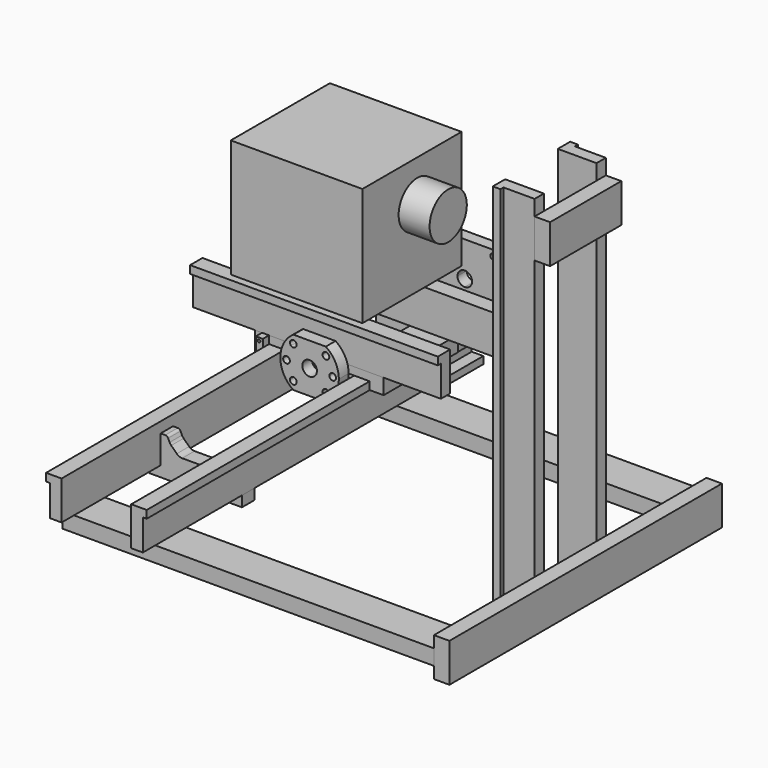
from build123d import *

# Parameters (mm, degrees)
F1_DEPTH       = 304.8
F3_DEPTH       = 76.2
F4_W           = 14.605
F4_H           = 6.35
F5_DEPTH       = 76.2
F7_DEPTH       = 25.4
F7_DEPTH_BACK  = 25.4
F9_DEPTH       = 3.175
F10_DEPTH      = 3.175
F12_DEPTH      = 6.35
F13_DEPTH      = 6.35
F15_DEPTH      = 6.35
F16_R          = 1.190625
F17_DEPTH      = 25.4
F18_DEPTH      = 25.4
F20_DEPTH      = 25.4
F23_DEPTH      = 10
F25_DEPTH      = 32
F27_DEPTH      = 25.4
F29_START      = 63.5
F28_R          = 6
F29_DEPTH      = 25
F30_DEPTH      = 50.8
F31_W          = 32.232244499
F31_H          = 34.175409925
F32_DEPTH      = 101.6
F34_DEPTH      = 50.8
F34_DEPTH_BACK = 152.4
F36_START      = -101.6
F36_DEPTH      = 12.7
F37_W          = 9.525
F37_H          = 5.95
F38_DEPTH      = 38.1
F39_W          = 31.75
F39_H          = 12.7
F40_DEPTH      = 304.8
F42_DEPTH      = 279.4
F44_DEPTH      = 304.8
F46_START      = 28.575
F46_DEPTH      = 9.525
F47_R          = 5.715
F48_DEPTH      = 3.175
F49_W          = 12.7
F49_H          = 31.75
F50_DEPTH      = 73.025
F51_W          = 107.9776808619
F51_H          = 96.8943238258
F52_DEPTH      = 101.6
F53_R          = 19.0804487929
F54_DEPTH      = 25.4


with BuildPart() as f1:
    # F0 (on Front) → F1 (new body)
    with BuildSketch(Plane.XZ):
        Polygon((-38.1, 25.4), (-38.1, 0), (-28.575, 0), (-28.575, 31.75), (-41.275, 31.75), (-41.275, 25.4), align=None)
    extrude(amount=F1_DEPTH)


with BuildPart() as f1b:
    # F0 (on Front) → F1, piece 2 (new body)
    with BuildSketch(Plane.XZ):
        Polygon((28.575, 31.75), (28.575, 0), (38.1, 0), (38.1, 25.4), (41.275, 25.4), (41.275, 31.75), align=None)
    extrude(amount=F1_DEPTH)


with BuildPart() as f3:
    # F2 (on face) → F3 (new body)
    with BuildSketch(Plane(origin=(0, 0, 0), x_dir=(-1, 0, 0), z_dir=(0, 1, 0))):
        Polygon((20.955, 31.75), (28.575, 31.75), (41.275, 31.75), (41.275, 25.4), (52.705, 25.4), (52.705, 38.1), (20.955, 38.1), align=None)
    extrude(amount=-F3_DEPTH)


with BuildPart() as f3b:
    # F2 (on face) → F3, piece 2 (new body)
    with BuildSketch(Plane(origin=(0, 0, 0), x_dir=(-1, 0, 0), z_dir=(0, 1, 0))):
        Polygon((-20.955, 31.75), (-20.955, 38.1), (-52.705, 38.1), (-52.705, 25.4), (-41.275, 25.4), (-41.275, 31.75), (-28.575, 31.75), align=None)
    extrude(amount=-F3_DEPTH)


with BuildPart() as f5:
    # F4 (on face) → F5 (new body)
    with BuildSketch(Plane(origin=(0, 0, 0), x_dir=(-1, 0, 0), z_dir=(0, 1, 0))):
        with Locations((45.4025, 22.225)):
            Rectangle(F4_W, F4_H)
    extrude(amount=-F5_DEPTH)


with BuildPart() as f7_tool:
    # F6 (on face) → F7 (new body, two sides)
    with BuildSketch(Plane(origin=(0, 0, 25.4), x_dir=(1, 0, 0), z_dir=(0, 0, -1))) as f7_sk:
        with BuildLine():
            ThreePointArc((-49.53, 6.35), (-51.1175, 4.7625), (-49.53, 3.175))
            Line((-49.53, 3.175), (-49.53, 6.35))
        make_face()
        with BuildLine():
            ThreePointArc((-49.53, 73.025), (-51.1175, 71.4375), (-49.53, 69.85))
            Line((-49.53, 69.85), (-49.53, 73.025))
        make_face()
        with BuildLine():
            Line((-49.53, 73.025), (-49.53, 69.85))
            ThreePointArc((-49.53, 69.85), (-48.4074679849, 70.3149679849), (-47.9425, 71.4375))
            ThreePointArc((-47.9425, 71.4375), (-48.4074679849, 72.5600320151), (-49.53, 73.025))
        make_face()
        with BuildLine():
            Line((-49.53, 6.35), (-49.53, 3.175))
            ThreePointArc((-49.53, 3.175), (-48.4074679849, 3.6399679849), (-47.9425, 4.7625))
            ThreePointArc((-47.9425, 4.7625), (-48.4074679849, 5.8850320151), (-49.53, 6.35))
        make_face()
    extrude(amount=-F7_DEPTH)
    extrude(f7_sk.sketch, amount=F7_DEPTH_BACK)


with BuildPart() as f3_1:
    add(f3.part)

    # F7: cut by f7_tool
    add(f7_tool.part, mode=Mode.SUBTRACT)

    # F11 (on face) → F12 (cut)
    with BuildSketch(Plane(origin=(0, 0, 25.4), x_dir=(1, 0, 0), z_dir=(0, 0, -1))):
        Polygon((-41.275, 0), (-41.275, 76.2), (-45.2059626353, 76.2), (-42.545, 0), align=None)
    extrude(amount=-F12_DEPTH, mode=Mode.SUBTRACT)


with BuildPart() as f5_1:
    add(f5.part)

    # F7: cut by f7_tool
    add(f7_tool.part, mode=Mode.SUBTRACT)

    # F8 (on face) → F9 (cut)
    with BuildSketch(Plane.YZ.offset(-38.1)):
        Polygon((0, 25.4), (-76.2, 25.4), (-76.2, 21.4690373647), (0, 24.13), align=None)
    extrude(amount=-F9_DEPTH, mode=Mode.SUBTRACT)


with BuildPart() as f10:
    # F8 (on face) → F10 (new body)
    with BuildSketch(Plane.YZ.offset(-38.1)):
        Polygon((0, 25.4), (-76.2, 25.4), (-76.2, 21.4690373647), (0, 24.13), align=None)
    extrude(amount=-F10_DEPTH)


with BuildPart() as f13:
    # F11 (on face) → F13 (new body)
    with BuildSketch(Plane(origin=(0, 0, 25.4), x_dir=(1, 0, 0), z_dir=(0, 0, -1))):
        Polygon((-41.275, 0), (-41.275, 76.2), (-45.2059626353, 76.2), (-42.545, 0), align=None)
    extrude(amount=-F13_DEPTH)


with BuildPart() as f15:
    # F14 (on face) → F15 (new body)
    with BuildSketch(Plane.XZ.offset(76.2)):
        Polygon((-41.275, 31.75), (-41.275, 38.1), (-46.99, 38.1), (-46.99, 25.4), (-45.2059626353, 25.4), (-45.2059626353, 31.75), align=None)
        Polygon((-41.275, 25.4), (-41.275, 31.75), (-45.2059626353, 31.75), (-45.2059626353, 25.4), (-46.99, 25.4), (-46.99, 19.05), (-38.1, 19.05), (-38.1, 25.4), align=None)
    extrude(amount=F15_DEPTH)


with BuildPart() as f17_tool:
    # F16 (on face) → F17 (new body)
    with BuildSketch(Plane.XZ.offset(82.55)):
        with Locations((-44.45, 35.56)):
            Circle(F16_R)
        with Locations((-44.45, 21.59)):
            Circle(F16_R)
    extrude(amount=-F17_DEPTH)


with BuildPart() as f3_2:
    add(f3_1.part)

    # F17: cut by f17_tool
    add(f17_tool.part, mode=Mode.SUBTRACT)

    # F19 (on face) → F20 (cut)
    with BuildSketch(Plane.XY.offset(38.1)):
        with BuildLine():
            Line((-25.7175, -4.7625), (-24.13, -4.7625))
            Line((-24.13, -4.7625), (-22.5425, -4.7625))
            ThreePointArc((-22.5425, -4.7625), (-24.13, -3.175), (-25.7175, -4.7625))
        make_face()
        with BuildLine():
            Line((-24.13, -6.35), (-24.13, -4.7625))
            Line((-24.13, -4.7625), (-25.7175, -4.7625))
            ThreePointArc((-25.7175, -4.7625), (-25.2525320151, -5.8850320151), (-24.13, -6.35))
        make_face()
        with BuildLine():
            Line((-22.5425, -4.7625), (-24.13, -4.7625))
            Line((-24.13, -4.7625), (-24.13, -6.35))
            ThreePointArc((-24.13, -6.35), (-23.0074679849, -5.8850320151), (-22.5425, -4.7625))
        make_face()
        with BuildLine():
            ThreePointArc((-22.5425, -71.4375), (-23.0074679849, -70.3149679849), (-24.13, -69.85))
            Line((-24.13, -69.85), (-24.13, -71.4375))
            Line((-24.13, -71.4375), (-22.5425, -71.4375))
        make_face()
        with BuildLine():
            Line((-24.13, -71.4375), (-24.13, -69.85))
            ThreePointArc((-24.13, -69.85), (-25.2525320151, -70.3149679849), (-25.7175, -71.4375))
            Line((-25.7175, -71.4375), (-24.13, -71.4375))
        make_face()
        with BuildLine():
            Line((-22.5425, -71.4375), (-24.13, -71.4375))
            Line((-24.13, -71.4375), (-25.7175, -71.4375))
            ThreePointArc((-25.7175, -71.4375), (-24.13, -73.025), (-22.5425, -71.4375))
        make_face()
    extrude(amount=-F20_DEPTH, mode=Mode.SUBTRACT)


with BuildPart() as f5_2:
    add(f5_1.part)

    # F17: cut by f17_tool
    add(f17_tool.part, mode=Mode.SUBTRACT)


with BuildPart() as f15_1:
    add(f15.part)

    # F17: cut by f17_tool
    add(f17_tool.part, mode=Mode.SUBTRACT)

    # F16 (on face) → F18 (cut)
    with BuildSketch(Plane.XZ.offset(82.55)):
        with Locations((-44.45, 35.56)):
            Circle(F16_R)
        with Locations((-44.45, 21.59)):
            Circle(F16_R)
        with BuildLine():
            Line((-44.053125, 28.575), (-41.671875, 28.575))
            ThreePointArc((-41.671875, 28.575), (-42.8625, 29.765625), (-44.053125, 28.575))
        make_face()
        with BuildLine():
            ThreePointArc((-44.053125, 28.575), (-42.8625, 27.384375), (-41.671875, 28.575))
            Line((-41.671875, 28.575), (-44.053125, 28.575))
        make_face()
        with BuildLine():
            ThreePointArc((-39.6875, 22.621875), (-38.8456009886, 22.9706009886), (-38.496875, 23.8125))
            ThreePointArc((-38.496875, 23.8125), (-38.8456009886, 24.6543990114), (-39.6875, 25.003125))
            Line((-39.6875, 25.003125), (-39.6875, 22.621875))
        make_face()
        with BuildLine():
            Line((-39.6875, 22.621875), (-39.6875, 25.003125))
            ThreePointArc((-39.6875, 25.003125), (-40.878125, 23.8125), (-39.6875, 22.621875))
        make_face()
    extrude(amount=-F18_DEPTH, mode=Mode.SUBTRACT)


with BuildPart() as f23:
    # F22 (on offset) → F23 (new body)
    with BuildSketch(Plane.XZ.offset(86.2)):
        with BuildLine():
            ThreePointArc((13.2664991614, 11.75), (21.1470562948, 20.4009026763), (24, 31.75))
            ThreePointArc((24, 31.75), (21.1470562948, 43.0990973237), (13.2664991614, 51.75))
            Line((13.2664991614, 51.75), (-13.2664991614, 51.75))
            ThreePointArc((-13.2664991614, 51.75), (-24, 31.75), (-13.2664991614, 11.75))
            Line((-13.2664991614, 11.75), (13.2664991614, 11.75))
        make_face()
    extrude(amount=-F23_DEPTH)

    # F24 (on face) → F25 (join)
    with BuildSketch(Plane(origin=(0, -76.2, 0), x_dir=(-1, 0, 0), z_dir=(0, 1, 0))):
        with BuildLine():
            ThreePointArc((14, 31.75), (9.8994949366, 41.6494949366), (0, 45.75))
            Line((0, 45.75), (0, 17.75))
            ThreePointArc((0, 17.75), (9.8994949366, 21.8505050634), (14, 31.75))
        make_face()
        with BuildLine():
            Line((0, 17.75), (0, 45.75))
            ThreePointArc((0, 45.75), (-14, 31.75), (0, 17.75))
        make_face()
    extrude(amount=F25_DEPTH)

    # F26 (on face) → F27 (cut)
    with BuildSketch(Plane(origin=(0, -76.2, 0), x_dir=(-1, 0, 0), z_dir=(0, 1, 0))):
        with BuildLine():
            ThreePointArc((-10.6406780721, 45.1406780721), (-10.824603754, 46.1294968594), (-11.3517781405, 46.9860471596))
            ThreePointArc((-11.3517781405, 46.9860471596), (-13.4350288425, 45.1850288425), (-15.2360471596, 43.1017781405))
            ThreePointArc((-15.2360471596, 43.1017781405), (-12.2753899906, 42.6269890509), (-10.6406780721, 45.1406780721))
        make_face()
        with BuildLine():
            ThreePointArc((-15.2360471596, 43.1017781405), (-13.4350288425, 45.1850288425), (-11.3517781405, 46.9860471596))
            ThreePointArc((-11.3517781405, 46.9860471596), (-15.3352217204, 47.0852217204), (-15.2360471596, 43.1017781405))
        make_face()
        with BuildLine():
            ThreePointArc((-18.8004315667, 29.0034070367), (-19, 31.75), (-18.8004315667, 34.4965929633))
            ThreePointArc((-18.8004315667, 34.4965929633), (-21.6872785389, 31.75), (-18.8004315667, 29.0034070367))
        make_face()
        with BuildLine():
            ThreePointArc((-18.8004315667, 29.0034070367), (-16.9449395651, 29.8544564333), (-16.1872785389, 31.75))
            ThreePointArc((-16.1872785389, 31.75), (-16.9449395651, 33.6455435667), (-18.8004315667, 34.4965929633))
            ThreePointArc((-18.8004315667, 34.4965929633), (-19, 31.75), (-18.8004315667, 29.0034070367))
        make_face()
        with BuildLine():
            ThreePointArc((-15.2360471596, 20.3982218595), (-15.3352217204, 16.4147782796), (-11.3517781405, 16.5139528404))
            ThreePointArc((-11.3517781405, 16.5139528404), (-13.4350288425, 18.3149711575), (-15.2360471596, 20.3982218595))
        make_face()
        with BuildLine():
            ThreePointArc((-15.2360471596, 20.3982218595), (-13.4350288425, 18.3149711575), (-11.3517781405, 16.5139528404))
            ThreePointArc((-11.3517781405, 16.5139528404), (-10.824603754, 17.3705031406), (-10.6406780721, 18.3593219279))
            ThreePointArc((-10.6406780721, 18.3593219279), (-12.2753899906, 20.8730109491), (-15.2360471596, 20.3982218595))
        make_face()
        with BuildLine():
            ThreePointArc((15.2360471596, 20.3982218595), (13.4350288425, 18.3149711575), (11.3517781405, 16.5139528404))
            ThreePointArc((11.3517781405, 16.5139528404), (14.3794968594, 15.7932476098), (16.1406780721, 18.3593219279))
            ThreePointArc((16.1406780721, 18.3593219279), (15.9043670933, 19.4746100094), (15.2360471596, 20.3982218595))
        make_face()
        with BuildLine():
            ThreePointArc((15.2360471596, 20.3982218595), (11.4461344238, 20.3038655762), (11.3517781405, 16.5139528404))
            ThreePointArc((11.3517781405, 16.5139528404), (13.4350288425, 18.3149711575), (15.2360471596, 20.3982218595))
        make_face()
        with BuildLine():
            ThreePointArc((19, 31.75), (18.9500422132, 33.126916888), (18.8004315667, 34.4965929633))
            ThreePointArc((18.8004315667, 34.4965929633), (16.1872785389, 31.75), (18.8004315667, 29.0034070367))
            ThreePointArc((18.8004315667, 29.0034070367), (18.9500422132, 30.373083112), (19, 31.75))
        make_face()
        with BuildLine():
            ThreePointArc((21.6872785389, 31.75), (20.8328221056, 33.7423389739), (18.8004315667, 34.4965929633))
            ThreePointArc((18.8004315667, 34.4965929633), (18.9500422132, 33.126916888), (19, 31.75))
            ThreePointArc((19, 31.75), (18.9500422132, 30.373083112), (18.8004315667, 29.0034070367))
            ThreePointArc((18.8004315667, 29.0034070367), (20.8328221056, 29.7576610261), (21.6872785389, 31.75))
        make_face()
        with BuildLine():
            ThreePointArc((16.1406780721, 45.1406780721), (14.3794968594, 47.7067523902), (11.3517781405, 46.9860471596))
            ThreePointArc((11.3517781405, 46.9860471596), (13.4350288425, 45.1850288425), (15.2360471596, 43.1017781405))
            ThreePointArc((15.2360471596, 43.1017781405), (15.9043670933, 44.0253899906), (16.1406780721, 45.1406780721))
        make_face()
        with BuildLine():
            ThreePointArc((15.2360471596, 43.1017781405), (13.4350288425, 45.1850288425), (11.3517781405, 46.9860471596))
            ThreePointArc((11.3517781405, 46.9860471596), (11.4461344238, 43.1961344238), (15.2360471596, 43.1017781405))
        make_face()
    extrude(amount=-F27_DEPTH, mode=Mode.SUBTRACT)

    # F28 (on face) → F30 (cut)
    with BuildSketch(Plane(origin=(0, -44.2, 0), x_dir=(-1, 0, 0), z_dir=(0, 1, 0))):
        with Locations((0, 31.75)):
            Circle(F28_R)
    extrude(amount=-F30_DEPTH, mode=Mode.SUBTRACT)

    # F31 (on face) → F32 (cut)
    with BuildSketch(Plane.XY.offset(51.75)):
        with Locations((-0.5382071249, -59.1122950375)):
            Rectangle(F31_W, F31_H)
    extrude(amount=-F32_DEPTH, mode=Mode.SUBTRACT)


with BuildPart() as f29:
    # F28 (on face) → F29 (new body)
    with BuildSketch(Plane(origin=(0, -44.2, 0), x_dir=(-1, 0, 0), z_dir=(0, 1, 0)).offset(F29_START)):
        with BuildLine():
            Line((-30, 39.25), (-30, 6.75))
            Line((-30, 6.75), (30, 6.75))
            Line((30, 6.75), (30, 39.25))
            Line((30, 39.25), (11.8215904175, 39.25))
            ThreePointArc((11.8215904175, 39.25), (13.4443717935, 35.6549797794), (14, 31.75))
            ThreePointArc((14, 31.75), (-3.9049797794, 18.3056282065), (-11.8215904175, 39.25))
            Line((-11.8215904175, 39.25), (-30, 39.25))
        make_face()
        with BuildLine():
            Line((11.8215904175, 39.25), (-11.8215904175, 39.25))
            ThreePointArc((-11.8215904175, 39.25), (-3.9049797794, 18.3056282065), (14, 31.75))
            ThreePointArc((14, 31.75), (13.4443717935, 35.6549797794), (11.8215904175, 39.25))
        make_face()
        with Locations((0, 31.75)):
            Circle(F28_R, mode=Mode.SUBTRACT)
    extrude(amount=F29_DEPTH)


with BuildPart() as f34:
    # F33 (on face) → F34 (new body, two sides)
    with BuildSketch(Plane(origin=(-52.705, 0, 0), x_dir=(0, -1, 0), z_dir=(-1, 0, 0))) as f34_sk:
        Polygon((79.375, 69.85), (66.675, 69.85), (66.675, 38.1), (76.2, 38.1), (76.2, 63.5), (79.375, 63.5), align=None)
    extrude(amount=F34_DEPTH)
    extrude(f34_sk.sketch, amount=-F34_DEPTH_BACK)


with BuildPart() as f34b:
    # F33 (on face) → F34, piece 2 (new body, two sides)
    with BuildSketch(Plane(origin=(-52.705, 0, 0), x_dir=(0, -1, 0), z_dir=(-1, 0, 0))) as f34_2_sk:
        Polygon((9.525, 38.1), (9.525, 69.85), (-3.175, 69.85), (-3.175, 63.5), (0, 63.5), (0, 38.1), align=None)
    extrude(amount=F34_DEPTH)
    extrude(f34_2_sk.sketch, amount=-F34_DEPTH_BACK)


with BuildPart() as f36:
    # F35 (on face) → F36 (new body)
    with BuildSketch(Plane.XZ.offset(304.8).offset(F36_START)):
        with BuildLine():
            Line((-28.575, 23.0663057628), (-28.575, 0))
            Line((-28.575, 0), (0, 0))
            Line((0, 0), (0, 10.8359847218))
            Line((0, 10.8359847218), (-10.9123596922, 10.8359847218))
            ThreePointArc((-10.9123596922, 10.8359847218), (-13.3188364584, 11.3096449109), (-15.3663046451, 12.6599628089))
            Line((-15.3663046451, 12.6599628089), (-19.9113620133, 17.1326400773))
            ThreePointArc((-19.9113620133, 17.1326400773), (-20.6495213407, 18.0029058247), (-21.2199982448, 18.9912366224))
            Line((-21.2199982448, 18.9912366224), (-22.4244490598, 21.59327591))
            ThreePointArc((-22.4244490598, 21.59327591), (-23.3617286636, 22.6665982865), (-24.7294815335, 23.0663057628))
            Line((-24.7294815335, 23.0663057628), (-28.575, 23.0663057628))
        make_face()
        with BuildLine():
            Line((0, 10.8359847218), (0, 0))
            Line((0, 0), (28.575, 0))
            Line((28.575, 0), (28.575, 23.0663057628))
            Line((28.575, 23.0663057628), (24.7294815335, 23.0663057628))
            ThreePointArc((24.7294815335, 23.0663057628), (23.3617286636, 22.6665982865), (22.4244490598, 21.59327591))
            Line((22.4244490598, 21.59327591), (21.2199982448, 18.9912366224))
            ThreePointArc((21.2199982448, 18.9912366224), (20.6495213407, 18.0029058247), (19.9113620133, 17.1326400773))
            Line((19.9113620133, 17.1326400773), (15.3663046451, 12.6599628089))
            ThreePointArc((15.3663046451, 12.6599628089), (13.3188364584, 11.3096449109), (10.9123596922, 10.8359847218))
            Line((10.9123596922, 10.8359847218), (0, 10.8359847218))
        make_face()
        Polygon((0, 0), (-28.575, 0), (-38.1, 0), (-38.1, -8.6836942372), (0, -8.6836942372), align=None)
        Polygon((28.575, 0), (0, 0), (0, -8.6836942372), (38.1, -8.6836942372), (38.1, 0), align=None)
    extrude(amount=-F36_DEPTH)


with BuildPart() as f38:
    # F37 (on face) → F38 (new body)
    with BuildSketch(Plane(origin=(0, 44.3, 0), x_dir=(-1, 0, 0), z_dir=(0, 1, 0))):
        Polygon((0, 6.75), (-28.575, 6.75), (-28.575, 0), (-28.575, -5.95), (0, -5.95), align=None)
        Polygon((28.575, 6.75), (0, 6.75), (0, -5.95), (28.575, -5.95), (28.575, 0), align=None)
        with Locations((-33.3375, -2.975)):
            Rectangle(F37_W, F37_H)
        with Locations((33.3375, -2.975)):
            Rectangle(F37_W, F37_H)
    extrude(amount=-F38_DEPTH)


with BuildPart() as f40:
    # F39 (on face) → F40 (new body)
    with BuildSketch(Plane(origin=(-38.1, 0, 0), x_dir=(0, -1, 0), z_dir=(-1, 0, 0))):
        with Locations((28.575, -6.35)):
            Rectangle(F39_W, F39_H)
    extrude(amount=-F40_DEPTH)


with BuildPart() as f40b:
    # F39 (on face) → F40, piece 2 (new body)
    with BuildSketch(Plane(origin=(-38.1, 0, 0), x_dir=(0, -1, 0), z_dir=(-1, 0, 0))):
        with Locations((276.225, -6.35)):
            Rectangle(F39_W, F39_H)
    extrude(amount=-F40_DEPTH)


with BuildPart() as f42:
    # F41 (on face) → F42 (new body)
    with BuildSketch(Plane.XZ.offset(292.1)):
        Polygon((266.7, -22.225), (279.4, -22.225), (279.4, 9.525), (266.7, 9.525), (266.7, 0), (266.7, -12.7), align=None)
    extrude(amount=-F42_DEPTH)


with BuildPart() as f44:
    # F43 (on face) → F44 (new body)
    with BuildSketch(Plane(origin=(0, 0, -22.225), x_dir=(1, 0, 0), z_dir=(0, 0, -1))):
        Polygon((266.7, 115.8875), (266.7, 125.4125), (234.95, 125.4125), (234.95, 112.7125), (241.3, 112.7125), (241.3, 115.8875), align=None)
    extrude(amount=-F44_DEPTH)


with BuildPart() as f44b:
    # F43 (on face) → F44, piece 2 (new body)
    with BuildSketch(Plane(origin=(0, 0, -22.225), x_dir=(1, 0, 0), z_dir=(0, 0, -1))):
        Polygon((234.95, 179.3875), (266.7, 179.3875), (266.7, 188.9125), (241.3, 188.9125), (241.3, 192.0875), (234.95, 192.0875), align=None)
    extrude(amount=-F44_DEPTH)


with BuildPart() as f46:
    # F45 (on face) → F46 (new body)
    with BuildSketch(Plane(origin=(0, 44.3, 0), x_dir=(-1, 0, 0), z_dir=(0, 1, 0)).offset(F46_START)):
        with BuildLine():
            ThreePointArc((-21.732233047, 10.017766953), (-21.1903011687, 9.2067085809), (-21, 8.25))
            Line((-21, 8.25), (0, 8.25))
            Line((0, 8.25), (0, 25.75))
            ThreePointArc((0, 25.75), (-2.2961005942, 26.2067228049), (-4.2426406871, 27.5073593129))
            Line((-4.2426406871, 27.5073593129), (-21.732233047, 10.017766953))
        make_face()
        with BuildLine():
            Line((0, 8.25), (-21, 8.25))
            ThreePointArc((-21, 8.25), (-21.1282917549, 7.459430585), (-21.5, 6.75))
            Line((-21.5, 6.75), (0, 6.75))
            Line((0, 6.75), (0, 8.25))
        make_face()
        with BuildLine():
            ThreePointArc((-25.5, 6.75), (-25.7360679775, 9.3680339887), (-23.5, 10.75))
            Line((-23.5, 10.75), (-23.5, 39.25))
            Line((-23.5, 39.25), (-28.5, 39.25))
            Line((-28.5, 39.25), (-28.5, 6.75))
            Line((-28.5, 6.75), (-25.5, 6.75))
        make_face()
        with BuildLine():
            Line((-23.5, 39.25), (-23.5, 10.75))
            ThreePointArc((-23.5, 10.75), (-22.5432914191, 10.5596988313), (-21.732233047, 10.017766953))
            Line((-21.732233047, 10.017766953), (-4.2426406871, 27.5073593129))
            ThreePointArc((-4.2426406871, 27.5073593129), (-5.5432771951, 34.0461005942), (0, 37.75))
            Line((0, 37.75), (0, 39.25))
            Line((0, 39.25), (-23.5, 39.25))
        make_face()
        with BuildLine():
            Line((0, 25.75), (0, 8.25))
            Line((0, 8.25), (21, 8.25))
            ThreePointArc((21, 8.25), (21.732233047, 10.017766953), (23.5, 10.75))
            Line((23.5, 10.75), (23.5, 39.25))
            Line((23.5, 39.25), (7.5, 39.25))
            Line((7.5, 39.25), (4.2426406871, 35.9926406871))
            ThreePointArc((4.2426406871, 35.9926406871), (5.5432771951, 34.0461005942), (6, 31.75))
            ThreePointArc((6, 31.75), (4.2426406871, 27.5073593129), (0, 25.75))
        make_face()
        with BuildLine():
            Line((21, 8.25), (0, 8.25))
            Line((0, 8.25), (0, 6.75))
            Line((0, 6.75), (21.5, 6.75))
            ThreePointArc((21.5, 6.75), (21.1282917549, 7.459430585), (21, 8.25))
        make_face()
        with BuildLine():
            Line((0, 6.75), (-21.5, 6.75))
            ThreePointArc((-21.5, 6.75), (-23.3227774498, 5.756289478), (-25.267766953, 6.482233047))
            Line((-25.267766953, 6.482233047), (-28.5, 3.25))
            Line((-28.5, 3.25), (0, 3.25))
            Line((0, 3.25), (0, 6.75))
        make_face()
        with BuildLine():
            Line((-28.5, 39.25), (-23.5, 39.25))
            Line((-23.5, 39.25), (-23.5, 52.75))
            ThreePointArc((-23.5, 52.75), (-25.267766953, 57.017766953), (-21, 55.25))
            Line((-21, 55.25), (0, 55.25))
            Line((0, 55.25), (21, 55.25))
            ThreePointArc((21, 55.25), (22.5432914191, 57.5596988313), (25.267766953, 57.017766953))
            Line((25.267766953, 57.017766953), (28.5, 60.25))
            Line((28.5, 60.25), (-28.5, 60.25))
            Line((-28.5, 60.25), (-28.5, 39.25))
        make_face()
        with BuildLine():
            Line((-23.5, 52.75), (-23.5, 39.25))
            Line((-23.5, 39.25), (0, 39.25))
            Line((0, 39.25), (0, 55.25))
            Line((0, 55.25), (-21, 55.25))
            ThreePointArc((-21, 55.25), (-21.732233047, 53.482233047), (-23.5, 52.75))
        make_face()
        with BuildLine():
            ThreePointArc((-25.267766953, 6.482233047), (-25.3886348875, 6.6119956466), (-25.5, 6.75))
            Line((-25.5, 6.75), (-28.5, 6.75))
            Line((-28.5, 6.75), (-28.5, 3.25))
            Line((-28.5, 3.25), (-25.267766953, 6.482233047))
        make_face()
        with BuildLine():
            Line((21.5, 6.75), (0, 6.75))
            Line((0, 6.75), (0, 3.25))
            Line((0, 3.25), (28.5, 3.25))
            Line((28.5, 3.25), (28.5, 6.75))
            Line((28.5, 6.75), (25.5, 6.75))
            ThreePointArc((25.5, 6.75), (23.5, 5.75), (21.5, 6.75))
        make_face()
        with BuildLine():
            Line((7.5, 39.25), (0, 39.25))
            Line((0, 39.25), (0, 37.75))
            ThreePointArc((0, 37.75), (2.2961005942, 37.2932771951), (4.2426406871, 35.9926406871))
            Line((4.2426406871, 35.9926406871), (7.5, 39.25))
        make_face()
        with BuildLine():
            Line((0, 55.25), (0, 39.25))
            Line((0, 39.25), (7.5, 39.25))
            Line((7.5, 39.25), (21.732233047, 53.482233047))
            ThreePointArc((21.732233047, 53.482233047), (21.1903011687, 54.2932914191), (21, 55.25))
            Line((21, 55.25), (0, 55.25))
        make_face()
        with BuildLine():
            Line((0, 3.25), (-28.5, 3.25))
            Line((-28.5, 3.25), (-28.5, -1.195))
            Line((-28.5, -1.195), (-15.875, -1.195))
            ThreePointArc((-15.875, -1.195), (-12.7, 1.98), (-9.525, -1.195))
            Line((-9.525, -1.195), (0, -1.195))
            Line((0, -1.195), (0, 3.25))
        make_face()
        with BuildLine():
            Line((23.5, 39.25), (23.5, 10.75))
            ThreePointArc((23.5, 10.75), (25.267766953, 10.017766953), (26, 8.25))
            ThreePointArc((26, 8.25), (25.8717082451, 7.459430585), (25.5, 6.75))
            Line((25.5, 6.75), (28.5, 6.75))
            Line((28.5, 6.75), (28.5, 39.25))
            Line((28.5, 39.25), (23.5, 39.25))
        make_face()
        with BuildLine():
            Line((28.5, 3.25), (0, 3.25))
            Line((0, 3.25), (0, -1.195))
            Line((0, -1.195), (9.525, -1.195))
            ThreePointArc((9.525, -1.195), (12.7, 1.98), (15.875, -1.195))
            Line((15.875, -1.195), (28.5, -1.195))
            Line((28.5, -1.195), (28.5, 3.25))
        make_face()
        with BuildLine():
            Line((21.732233047, 53.482233047), (7.5, 39.25))
            Line((7.5, 39.25), (23.5, 39.25))
            Line((23.5, 39.25), (23.5, 52.75))
            ThreePointArc((23.5, 52.75), (22.5432914191, 52.9403011687), (21.732233047, 53.482233047))
        make_face()
        with BuildLine():
            Line((-15.875, -1.195), (-28.5, -1.195))
            Line((-28.5, -1.195), (-28.5, -5.64))
            Line((-28.5, -5.64), (0, -5.64))
            Line((0, -5.64), (0, -1.195))
            Line((0, -1.195), (-9.525, -1.195))
            ThreePointArc((-9.525, -1.195), (-12.7, -4.37), (-15.875, -1.195))
        make_face()
        with BuildLine():
            Line((23.5, 52.75), (23.5, 39.25))
            Line((23.5, 39.25), (28.5, 39.25))
            Line((28.5, 39.25), (28.5, 60.25))
            Line((28.5, 60.25), (25.267766953, 57.017766953))
            ThreePointArc((25.267766953, 57.017766953), (25.8096988313, 56.2067085809), (26, 55.25))
            ThreePointArc((26, 55.25), (25.267766953, 53.482233047), (23.5, 52.75))
        make_face()
        with BuildLine():
            Line((9.525, -1.195), (0, -1.195))
            Line((0, -1.195), (0, -5.64))
            Line((0, -5.64), (28.5, -5.64))
            Line((28.5, -5.64), (28.5, -1.195))
            Line((28.5, -1.195), (15.875, -1.195))
            ThreePointArc((15.875, -1.195), (12.7, -4.37), (9.525, -1.195))
        make_face()
    extrude(amount=F46_DEPTH)

    # F47 (on face) → F48 (cut)
    with BuildSketch(Plane(origin=(0, 82.4, 0), x_dir=(-1, 0, 0), z_dir=(0, 1, 0))):
        with Locations((-12.7, -1.195)):
            Circle(F47_R)
        with Locations((12.7, -1.195)):
            Circle(F47_R)
    extrude(amount=-F48_DEPTH, mode=Mode.SUBTRACT)


with BuildPart() as f50:
    # F49 (on face) → F50 (new body)
    with BuildSketch(Plane(origin=(0, -115.8875, 0), x_dir=(-1, 0, 0), z_dir=(0, 1, 0))):
        with Locations((-273.05, 254)):
            Rectangle(F49_W, F49_H)
    extrude(amount=-F50_DEPTH)


with BuildPart() as f52:
    # F51 (on Front) → F52 (new body)
    with BuildSketch(Plane.XZ):
        with Locations((1.6513057053, 137.138530612)):
            Rectangle(F51_W, F51_H)
    extrude(amount=F52_DEPTH)

    # F53 (on face) → F54 (join)
    with BuildSketch(Plane.YZ.offset(55.6401461363)):
        with Locations((-45.4014539719, 151.7196297646)):
            Circle(F53_R)
    extrude(amount=F54_DEPTH)


solid = Compound([f1.part, f1b.part, f3b.part, f10.part, f13.part, f3_2.part, f5_2.part, f15_1.part, f23.part, f29.part, f34.part, f34b.part, f36.part, f38.part, f40.part, f40b.part, f42.part, f44.part, f44b.part, f46.part, f50.part, f52.part])
